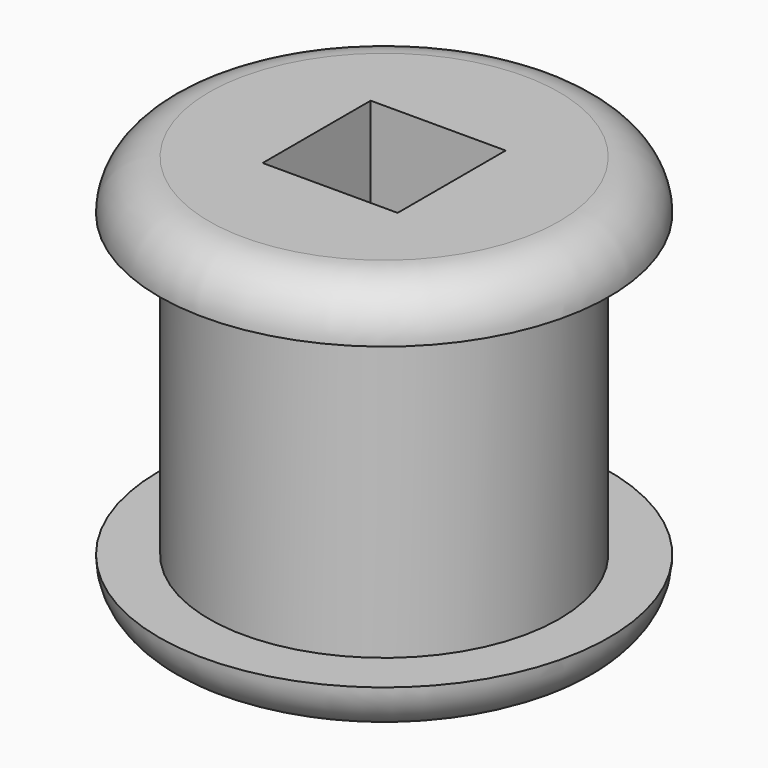
from build123d import *

# Parameters (mm, degrees)
F2_W     = 3.429
F2_H     = 3.429
F3_DEPTH = 25.4
F4_R     = 1.26999
F5_R     = 1.26999


# Not quite as in the source:
# - a fillet or chamfer is up to 0.001 mm smaller than in the source, because OpenCascade refuses the exact size


with BuildPart() as f1:
    # F0 (on Front) → F1 (revolve)
    with BuildSketch(Plane.XZ):
        Polygon((-1.27, 0), (0, 0), (4.445, 0), (4.445, 10.16), (0, 10.16), (-1.27, 10.16), (-1.27, 8.89), (0, 8.89), (0, 1.27), (-1.27, 1.27), align=None)
    revolve(axis=Axis((4.445, 0, 5.08), (0, 0, -1)))

    # F2 (on face) → F3 (cut)
    with BuildSketch(Plane(origin=(0, 0, 0), x_dir=(1, 0, 0), z_dir=(0, 0, -1))):
        with Locations((4.445, 0)):
            Rectangle(F2_W, F2_H)
    extrude(amount=-F3_DEPTH, mode=Mode.SUBTRACT)

    # F4 (radius 1.27 in the source; OpenCascade refuses exactly that, so slightly less here)
    f4_edges = [f1.edges().sort_by_distance(p)[0] for p in [
        (10.16, 0, 0),
    ]]
    fillet(f4_edges, radius=F4_R)

    # F5 (radius 1.27 in the source; OpenCascade refuses exactly that, so slightly less here)
    f5_edges = [f1.edges().sort_by_distance(p)[0] for p in [
        (10.16, 0, 10.16),
    ]]
    fillet(f5_edges, radius=F5_R)


solid = f1.part
